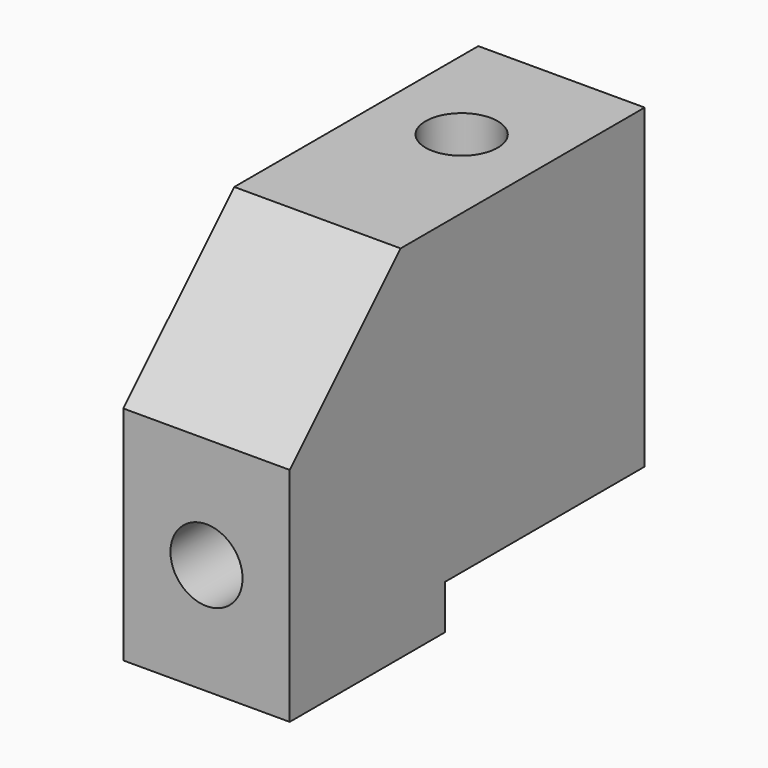
from build123d import *

# Parameters (mm, degrees)
F1_DEPTH = 6
F4_D     = 2.6
F5_D     = 2.6
F5_DEPTH = 9
F5_TIP   = 0.7811188047


with BuildPart() as f1:
    # F0 (on Right) → F1 (new body)
    with BuildSketch(Plane.YZ):
        Polygon((0, 8), (0, 0), (7, 0), (7, 1.6), (16, 1.6), (16, 13), (5, 13), align=None)
    extrude(amount=F1_DEPTH)

    # F4 (through all)
    with Locations(Plane.XY.offset(13)):
        with Locations((3, 11.5)):
            Hole(F4_D / 2)

    # F5
    with Locations(Plane.XZ):
        with Locations((3, 4)):
            Hole(F5_D / 2, depth=F5_DEPTH)
            with Locations((0, 0, -(F5_DEPTH + F5_TIP / 2))):  # 118° drill point
                Cone(0, F5_D / 2, F5_TIP, mode=Mode.SUBTRACT)


solid = f1.part
